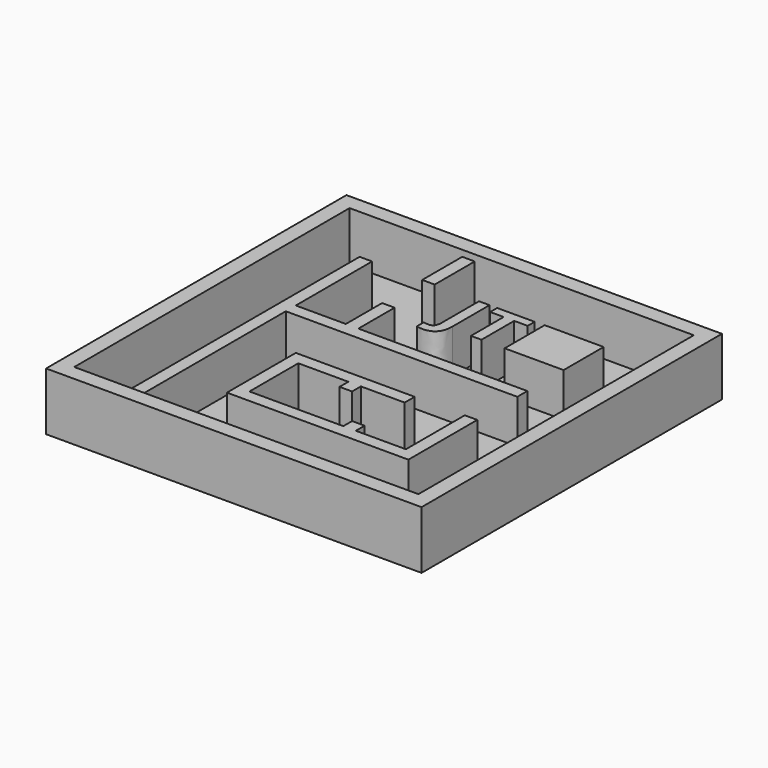
from build123d import *

# Parameters (mm, degrees)
F0_W         = 38.1
F0_H         = 38.1
F1_DEPTH     = 0.79375
F2_W         = 38.1
F2_H         = 38.1
F2_W_2       = 34.925
F2_H_2       = 34.925
F3_DEPTH     = 5.08
F4_W         = 1.27
F4_H         = 5.08
F4_W_2       = 5.9844940627
F5_DEPTH     = 4.445
F6_R         = 1.27
F7_DEPTH     = 0.396875
F6_TEXT_SIZE = 7.0555555556
F8_DEPTH     = 4.445


# Not quite as in the source:
# - Text() gives the source's letters only with a copy of the font that has no kerning and outlines rounded to 1/6400 em; it was checked with that copy


with BuildPart() as f1:
    # F0 (on Top) → F1 (new body)
    with BuildSketch(Plane.XY):
        with Locations((-0.0905027288, 0.180143863)):
            Rectangle(F0_W, F0_H)
    extrude(amount=F1_DEPTH)

    # F2 (on face) → F3 (join)
    with BuildSketch(Plane.XY.offset(0.79375)):
        with Locations((-0.0905027288, 0.180143863)):
            Rectangle(F2_W, F2_H)
        with Locations((-0.0905027288, 0.180143863)):
            Rectangle(F2_W_2, F2_H_2, mode=Mode.SUBTRACT)
    extrude(amount=F3_DEPTH)

    # F4 (on face) → F5 (join)
    with BuildSketch(Plane.XY.offset(0.79375)):
        Polygon((-11.2030027288, 12.562643863), (-12.4730027288, 12.562643863), (-12.4730027288, -17.282356137), (-11.2030027288, -17.282356137), (-11.2030027288, 1.612070134), (-6.1230027288, 1.612070134), (-4.8530027288, 1.612070134), (12.2919972712, 1.612070134), (12.2919972712, 2.882070134), (-4.8530027288, 2.882070134), (-4.8530027288, 7.482643863), (-6.1230027288, 7.482643863), (-6.1230027288, 2.882070134), (-11.2030027288, 2.882070134), align=None)
        Polygon((-4.8530027288, -3.467929866), (-6.1230027288, -3.467929866), (-6.1230027288, -12.202356137), (-4.8530027288, -12.202356137), (12.2919972712, -12.202356137), (12.2919972712, -10.932356137), (12.2919972712, -3.467929866), (11.0219972712, -3.467929866), (11.0219972712, -10.932356137), (5.9419972712, -10.932356137), (5.9419972712, -9.817929866), (4.6719972712, -9.817929866), (4.6719972712, -10.932356137), (-4.8530027288, -10.932356137), (-4.8530027288, -4.737929866), (0.2269972712, -4.737929866), (0.2269972712, -5.852356137), (1.4969972712, -5.852356137), (1.4969972712, -4.737929866), (5.9419972712, -4.737929866), (5.9419972712, -3.467929866), align=None)
        with Locations((-5.4880027288, 15.102643863)):
            Rectangle(F4_W, F4_H)
        with Locations((9.2997502399, 10.022643863)):
            Rectangle(F4_W_2, F4_H)
    extrude(amount=F5_DEPTH)

    # F6 (on face) → F7 (cut)
    with BuildSketch(Plane.XY.offset(0.79375)):
        with Locations((-2.0784543865, -8.1990678996)):
            Circle(F6_R)
        with Locations((-15.0240743356, -14.4402323841)):
            Circle(F6_R)
    extrude(amount=-F7_DEPTH, mode=Mode.SUBTRACT)

    # F6 (on face) → F8 (join)
    with BuildSketch(Plane.XY.offset(0.79375)):
        with Locations((-0.9542068609, 7.482643863)):
            Text('JT', F6_TEXT_SIZE, font='Open Sans', font_style=FontStyle.BOLD, text_align=(TextAlign.LEFT, TextAlign.BOTTOM))
    extrude(amount=F8_DEPTH)


solid = f1.part
